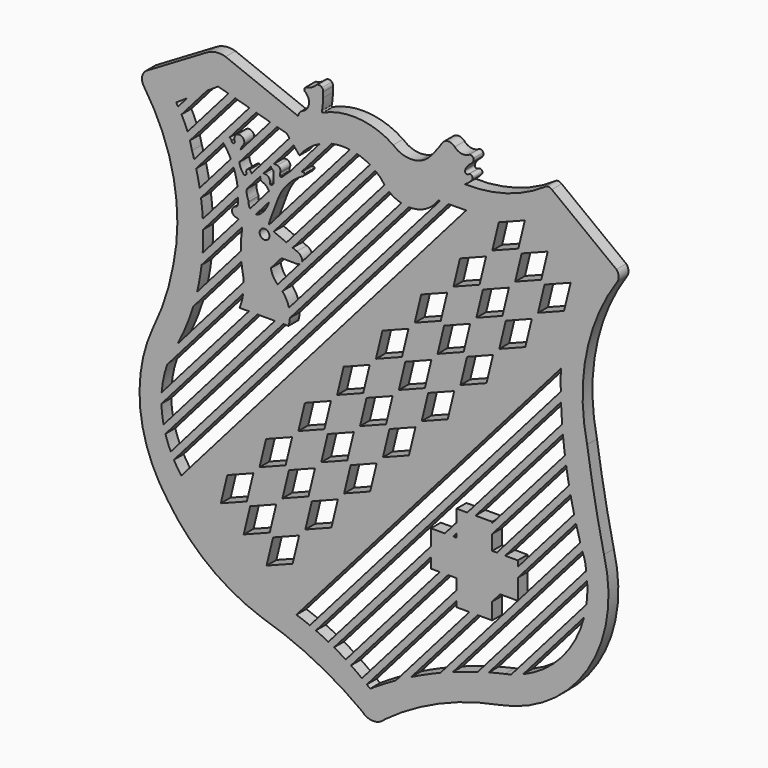
from build123d import *

# Parameters (mm, degrees)
F0_R     = 0.3088668402
F1_DEPTH = 0.77
F2_SCALE = 2.61


# Not quite as in the source:
# - ends of sketch curves that miss each other by under 0.0002 mm in the source are joined


with BuildPart() as f1:
    # F0 (on Front) → F1 (new body)
    with BuildSketch(Plane.XZ):
        with BuildLine():
            Line((-10.9450528398, 8.238459006), (-14.7752109915, 5.9727313928))
            ThreePointArc((-14.7752109915, 5.9727313928), (-15.0157556415, 5.5361442766), (-14.8831028491, 5.0556515343))
            ThreePointArc((-14.8831028491, 5.0556515343), (-13.0285590849, 0.6195466195), (-13.0580402911, -4.1885185055))
            ThreePointArc((-13.0580402911, -4.1885185055), (-13.5568964145, -6.159584329), (-14.3210859969, -8.0437213182))
            ThreePointArc((-14.3210859969, -8.0437213182), (-15.1281021661, -12.7854152226), (-13.4050389752, -17.276071012))
            ThreePointArc((-13.4050389752, -17.276071012), (-10.8401080038, -20.0274931211), (-7.5306314975, -21.8153856695))
            ThreePointArc((-7.5306314975, -21.8153856695), (-4.2408430264, -23.1051475942), (-1.226167893, -24.9484945089))
            ThreePointArc((-1.226167893, -24.9484945089), (-0.5230431925, -25.2671373593), (0.180081508, -24.9484945089))
            ThreePointArc((0.180081508, -24.9484945089), (3.5801467972, -22.973795852), (7.3375348002, -21.8153856695))
            ThreePointArc((7.3375348002, -21.8153856695), (12.9195911311, -18.040178348), (13.9394840226, -11.3789951429))
            ThreePointArc((13.9394840226, -11.3789951429), (13.3587393158, -8.5258534115), (12.8830319769, -5.6533310562))
            ThreePointArc((12.8830319769, -5.6533310562), (12.826516045, -0.6803487089), (14.7480200976, 3.9067603648))
            ThreePointArc((14.7480200976, 3.9067603648), (14.8574048465, 4.2653018977), (14.7159444168, 4.6124416403))
            Line((14.7159444168, 4.6124416403), (10.6676835567, 7.7041857041))
            ThreePointArc((10.6676835567, 7.7041857041), (10.4508174999, 7.789802789), (10.2339514432, 7.7041857041))
            ThreePointArc((10.2339514432, 7.7041857041), (7.8431577076, 6.5715789898), (5.2206409829, 6.223586627))
            Line((5.2206409829, 6.223586627), (5.2057327849, 6.2239474028))
            ThreePointArc((5.2057327849, 6.2239474028), (5.2128688846, 6.2275017661), (5.2199811789, 6.2311035281))
            ThreePointArc((5.2199811789, 6.2311035281), (5.4576814871, 6.3909100368), (5.6506660767, 6.6025618852))
            ThreePointArc((5.6506660767, 6.6025618852), (5.666017401, 6.8296722857), (5.438990331, 6.8450179774))
            ThreePointArc((5.438990331, 6.8450179774), (5.2774498824, 6.8438940146), (5.2317598398, 6.9988423926))
            ThreePointArc((5.2317598398, 6.9988423926), (5.3413345105, 7.2160766667), (5.5031483062, 7.39777321))
            ThreePointArc((5.5031483062, 7.39777321), (5.6486132018, 7.5233006308), (5.7621701773, 7.6782908968))
            ThreePointArc((5.7621701773, 7.6782908968), (5.7744494367, 7.7563651745), (5.7568072409, 7.8334049433))
            ThreePointArc((5.7568072409, 7.8334049433), (5.6517282464, 7.9393365939), (5.5027715738, 7.9479979673))
            ThreePointArc((5.5027715738, 7.9479979673), (5.0188791458, 7.8403294095), (4.5830812305, 8.0766016617))
            ThreePointArc((4.5830812305, 8.0766016617), (4.14755377, 8.2479055445), (3.7629532162, 7.9812379554))
            ThreePointArc((3.7629532162, 7.9812379554), (3.4440060295, 7.5359280459), (3.0954068061, 7.1134273894))
            ThreePointArc((3.0954068061, 7.1134273894), (2.7632061359, 6.8020403745), (2.3577139174, 6.5949287643))
            ThreePointArc((2.3577139174, 6.5949287643), (1.4977198293, 6.5400653755), (0.7303855964, 6.9322362542))
            ThreePointArc((0.7303855964, 6.9322362542), (-1.4116971773, 7.6752869671), (-3.6468112376, 7.2946189903))
            ThreePointArc((-3.6468112376, 7.2946189903), (-3.7266554182, 7.2894142265), (-3.7329988554, 7.369176019))
            ThreePointArc((-3.7329988554, 7.369176019), (-3.6863749188, 7.7291436193), (-3.6669184756, 8.0915962529))
            ThreePointArc((-3.6669184756, 8.0915962529), (-3.6669370542, 8.2476662803), (-3.6719986238, 8.4036542103))
            ThreePointArc((-3.6719986238, 8.4036542103), (-3.6744007516, 8.529985654), (-3.7354342298, 8.6406216267))
            ThreePointArc((-3.7354342298, 8.6406216267), (-3.9275077773, 8.7250033825), (-4.120208323, 8.6420634761))
            ThreePointArc((-4.120208323, 8.6420634761), (-4.3903821308, 8.4401648063), (-4.7114635818, 8.3368998021))
            ThreePointArc((-4.7114635818, 8.3368998021), (-4.8381657863, 8.2245188579), (-4.7927666456, 8.0613568425))
            ThreePointArc((-4.7927666456, 8.0613568425), (-4.5483256085, 7.5070030075), (-4.8736855388, 6.9959252141))
            ThreePointArc((-4.8736855388, 6.9959252141), (-5.1085754677, 6.8393309853), (-5.2295372828, 6.5842559561))
            Line((-5.2295372828, 6.5842559561), (-9.7806490958, 8.3812242374))
            ThreePointArc((-9.7806490958, 8.3812242374), (-10.3777742193, 8.4315567602), (-10.9450528398, 8.238459006))
        make_face()
        Polygon((-5.5775461902, -18.2294403803), (-7.2106110116, -18.8645213511), (-6.8023452719, -17.1747529548), (-5.1692804505, -16.5396719839), align=None, mode=Mode.SUBTRACT)
        Polygon((-8.4461733818, -15.7241220544), (-10.0792382032, -16.3592030252), (-9.6709724635, -14.6694346289), (-8.0379076422, -14.0343536581), align=None, mode=Mode.SUBTRACT)
        with BuildLine():
            ThreePointArc((-13.6667065556, -13.1795461358), (-13.7572572831, -12.6297862933), (-13.7985303908, -12.0741498572))
            Line((-13.7985303908, -12.0741498572), (-7.7867736006, -5.1905978471))
            Line((-7.7867736006, -5.1905978471), (-6.6895508588, -5.1905978471))
            Line((-6.6895508588, -5.1905978471), (-13.6667065556, -13.1795461358))
        make_face(mode=Mode.SUBTRACT)
        Polygon((-7.011859786, -16.9767812173), (-8.6449246074, -17.6118621881), (-8.2366588677, -15.9220937918), (-6.6035940463, -15.287012821), align=None, mode=Mode.SUBTRACT)
        Polygon((-4.5809357093, -14.1933365607), (-6.2140005306, -14.8284175315), (-5.805734791, -13.1386491352), (-4.1726699696, -12.5035681644), align=None, mode=Mode.SUBTRACT)
        Polygon((-3.1466221135, -15.4459957236), (-4.7796869348, -16.0810766945), (-4.3714211952, -14.3913082981), (-2.7383563738, -13.7562273273), align=None, mode=Mode.SUBTRACT)
        Polygon((-6.0152493051, -12.9406773977), (-7.6483141265, -13.5757583686), (-7.2400483868, -11.8859899723), (-5.6069835654, -11.2509090014), align=None, mode=Mode.SUBTRACT)
        Polygon((-3.5843252284, -10.1572327411), (-5.2173900497, -10.7923137119), (-4.80912431, -9.1025453156), (-3.1760594887, -8.4674643448), align=None, mode=Mode.SUBTRACT)
        Polygon((-2.1500116325, -11.4098919041), (-3.7830764539, -12.0449728749), (-3.3748107142, -10.3552044786), (-1.7417458929, -9.7201235077), align=None, mode=Mode.SUBTRACT)
        Polygon((-0.7156980367, -12.662551067), (-2.3487628581, -13.2976320378), (-1.9404971184, -11.6078636415), (-0.307432297, -10.9727826707), align=None, mode=Mode.SUBTRACT)
        with BuildLine():
            ThreePointArc((-1.2333306094, -23.1370316943), (-1.571815927, -22.8880537555), (-1.9174369369, -22.6490800294))
            Line((-1.9174369369, -22.6490800294), (4.1664697033, -15.6829153552))
            Line((4.1664697033, -15.6829153552), (4.6998463428, -15.6829153552))
            Line((4.6998463428, -15.6829153552), (4.6998463428, -16.3434547816))
            Line((4.6998463428, -16.3434547816), (-1.2333306094, -23.1370316943))
        make_face(mode=Mode.SUBTRACT)
        with BuildLine():
            ThreePointArc((0.8920551407, -22.5697107783), (0.0769750695, -23.0424218327), (-0.7199500254, -23.5451361219))
            ThreePointArc((-0.7199500254, -23.5451361219), (-0.8217137816, -23.4611676966), (-0.9242442608, -23.3781372242))
            Line((-0.9242442608, -23.3781372242), (4.6998463428, -16.9384688328))
            Line((4.6998463428, -16.9384688328), (4.6998463428, -17.2902317473))
            Line((4.6998463428, -17.2902317473), (5.5028932468, -17.2902317473))
            Line((5.5028932468, -17.2902317473), (0.8920551407, -22.5697107783))
        make_face(mode=Mode.SUBTRACT)
        with BuildLine():
            Line((3.6468136075, -15.6829153552), (-2.2488664966, -22.4335578124))
            ThreePointArc((-2.2488664966, -22.4335578124), (-2.6119716601, -22.2119287852), (-2.9814786804, -22.0011460831))
            Line((-2.9814786804, -22.0011460831), (3.0925299507, -15.0463147783))
            Line((3.0925299507, -15.0463147783), (3.0925299507, -15.6829153552))
            Line((3.0925299507, -15.6829153552), (3.6468136075, -15.6829153552))
        make_face(mode=Mode.SUBTRACT)
        with BuildLine():
            Line((8.5365600495, -15.6829153552), (3.6889344902, -21.2335195841))
            ThreePointArc((3.6889344902, -21.2335195841), (2.7640681021, -21.6292399404), (1.8556529669, -22.061390815))
            Line((1.8556529669, -22.061390815), (6.0225493426, -17.2902317473))
            Line((6.0225493426, -17.2902317473), (6.9292436575, -17.2902317473))
            Line((6.9292436575, -17.2902317473), (6.9292436575, -16.2520531098))
            Line((6.9292436575, -16.2520531098), (7.4263006647, -15.6829153552))
            Line((7.4263006647, -15.6829153552), (8.5365600495, -15.6829153552))
        make_face(mode=Mode.SUBTRACT)
        with BuildLine():
            ThreePointArc((12.6890300152, -15.2558443111), (11.2945144522, -17.8938182952), (8.8682408565, -19.6307054059))
            Line((8.8682408565, -19.6307054059), (12.6890300152, -15.2558443111))
        make_face(mode=Mode.SUBTRACT)
        with BuildLine():
            Line((-4.1196529229, -21.4380949639), (11.2479575195, -3.8419497037))
            ThreePointArc((11.2479575195, -3.8419497037), (11.2764123646, -4.4385333427), (11.3167625343, -5.0344306328))
            Line((11.3167625343, -5.0344306328), (5.3676957448, -11.8462016484))
            Line((5.3676957448, -11.8462016484), (4.6998463428, -11.8462016484))
            Line((4.6998463428, -11.8462016484), (4.6998463428, -12.6108992658))
            Line((4.6998463428, -12.6108992658), (3.9639444228, -13.4535180405))
            Line((3.9639444228, -13.4535180405), (3.0925299507, -13.4535180405))
            Line((3.0925299507, -13.4535180405), (3.0925299507, -14.4513007271))
            Line((3.0925299507, -14.4513007271), (-3.3360950096, -21.8121730663))
            ThreePointArc((-3.3360950096, -21.8121730663), (-3.7250476456, -21.6192138986), (-4.1196529229, -21.4380949639))
        make_face(mode=Mode.SUBTRACT)
        Polygon((4.6998463428, -13.4535180405), (4.4836005186, -13.4535180405), (4.6998463428, -13.2059133171), align=None, mode=Mode.SUBTRACT)
        with BuildLine():
            Line((-5.3373983951, -20.9661541004), (11.2354560879, -1.9899862731))
            ThreePointArc((11.2354560879, -1.9899862731), (11.2268252487, -2.6277027287), (11.2317807175, -3.2654583342))
            Line((11.2317807175, -3.2654583342), (-4.4989278267, -21.2773563861))
            ThreePointArc((-4.4989278267, -21.2773563861), (-4.9157411664, -21.1152298116), (-5.3373983952, -20.9661541004))
        make_face(mode=Mode.SUBTRACT)
        Polygon((1.71522604, -9.8791064104), (0.0821612187, -10.5141873812), (0.4904269583, -8.8244189849), (2.1234917797, -8.1893380141), align=None, mode=Mode.SUBTRACT)
        with BuildLine():
            Line((6.0321875111, -20.4167373638), (4.4722335106, -20.9316444673))
            Line((4.4722335106, -20.9316444673), (12.5894441115, -11.6373161539))
            ThreePointArc((12.5894441115, -11.6373161539), (12.7448209703, -12.1294752601), (12.8245471129, -12.6393833853))
            Line((12.8245471129, -12.6393833853), (6.0321875111, -20.4167373638))
        make_face(mode=Mode.SUBTRACT)
        with BuildLine():
            ThreePointArc((8.1273773746, -19.8839911925), (7.9218788322, -19.9370827443), (7.7147563921, -19.9834363697))
            ThreePointArc((7.7147563921, -19.9834363697), (7.2158699773, -20.0991111557), (6.7194254717, -20.2248536063))
            Line((6.7194254717, -20.2248536063), (12.8830319769, -13.1674313871))
            ThreePointArc((12.8830319769, -13.1674313871), (12.895286878, -13.8286196949), (12.8402937453, -14.4876310122))
            Line((12.8402937453, -14.4876310122), (8.1273773746, -19.8839911925))
        make_face(mode=Mode.SUBTRACT)
        with BuildLine():
            Line((8.5365600495, -14.4116516486), (12.1862088162, -10.2327488784))
            ThreePointArc((12.1862088162, -10.2327488784), (12.315988426, -10.716281355), (12.453835442, -11.1975760705))
            Line((12.453835442, -11.1975760705), (8.5464982905, -15.6715359198))
            Line((8.5464982905, -15.6715359198), (8.5365600495, -14.4116516486))
        make_face(mode=Mode.SUBTRACT)
        with BuildLine():
            Line((7.74343148, -13.4535180405), (11.8433498423, -8.7590498063))
            ThreePointArc((11.8433498423, -8.7590498063), (11.9524009398, -9.2657852479), (12.0702086391, -9.770556776))
            Line((12.0702086391, -9.770556776), (8.5365600495, -13.8166375973))
            Line((8.5365600495, -13.8166375973), (8.5365600495, -13.4535180405))
            Line((8.5365600495, -13.4535180405), (7.74343148, -13.4535180405))
        make_face(mode=Mode.SUBTRACT)
        with BuildLine():
            Line((5.8873518406, -11.8462016484), (11.3637776151, -5.5756117089))
            ThreePointArc((11.3637776151, -5.5756117089), (11.4231257209, -6.1378278281), (11.4930792726, -6.6988230715))
            Line((11.4930792726, -6.6988230715), (6.9292436575, -11.9244835428))
            Line((6.9292436575, -11.9244835428), (6.9292436575, -11.8462016484))
            Line((6.9292436575, -11.8462016484), (5.8873518406, -11.8462016484))
        make_face(mode=Mode.SUBTRACT)
        with BuildLine():
            Line((6.9292436575, -12.5194975941), (11.5669223234, -7.2146120887))
            ThreePointArc((11.5669223234, -7.2146120887), (11.6524503811, -7.7450187223), (11.7474826057, -8.2738051838))
            Line((11.7474826058, -8.2738051838), (7.2237753842, -13.4535180405))
            Line((7.2237753842, -13.4535180405), (6.9292436575, -13.4535180405))
            Line((6.9292436575, -13.4535180405), (6.9292436575, -12.5194975941))
        make_face(mode=Mode.SUBTRACT)
        with BuildLine():
            ThreePointArc((-13.7858184066, -11.4496532401), (-13.6697387353, -10.6130173489), (-13.4420062366, -9.7996465765))
            Line((-13.4420062366, -9.7996465765), (-8.677906045, -4.3446801508))
            ThreePointArc((-8.677906045, -4.3446801508), (-8.7616198951, -4.7738576747), (-8.8940169662, -5.1905978471))
            Line((-8.8940169662, -5.1905978471), (-8.3194663395, -5.1905978471))
            Line((-8.3194663395, -5.1905978471), (-13.7858184066, -11.4496532401))
        make_face(mode=Mode.SUBTRACT)
        with BuildLine():
            Line((-8.6455751358, -3.6977195694), (-12.77777931, -8.4291555443))
            ThreePointArc((-12.77777931, -8.4291555443), (-12.2372024074, -7.2658242862), (-11.8043741052, -6.0582553795))
            Line((-11.8043741052, -6.0582553795), (-8.7869307107, -2.6032372762))
            ThreePointArc((-8.7869307107, -2.6032372762), (-8.7410410218, -2.9675427525), (-8.6765894666, -3.32902628))
            ThreePointArc((-8.6765894666, -3.32902628), (-8.656598502, -3.5129957493), (-8.6455751358, -3.6977195694))
        make_face(mode=Mode.SUBTRACT)
        with BuildLine():
            Line((-8.821167106, -2.0324972603), (-11.5625482211, -5.1714198987))
            ThreePointArc((-11.5625482211, -5.1714198987), (-11.3989515702, -4.3856405891), (-11.2802423771, -3.5918389041))
            Line((-11.2802423771, -3.5918389041), (-8.7387201501, -0.6817577008))
            ThreePointArc((-8.7387201501, -0.6817577008), (-8.7348520945, -0.7841341496), (-8.7522082031, -0.8851027815))
            ThreePointArc((-8.7522082031, -0.8851027815), (-8.8096825125, -1.45741802), (-8.821167106, -2.0324972603))
        make_face(mode=Mode.SUBTRACT)
        with BuildLine():
            Line((-8.9664455479, -0.3325655051), (-11.2144849522, -2.906604459))
            ThreePointArc((-11.2144849522, -2.906604459), (-11.1831679624, -2.2599358856), (-11.1815104167, -1.6125115655))
            Line((-11.1815104167, -1.6125115655), (-8.9905998315, 0.8961140307))
            ThreePointArc((-8.9905998315, 0.8961140307), (-8.9944051774, 0.699791789), (-9.0069510043, 0.5038338713))
            ThreePointArc((-9.0069510043, 0.5038338713), (-9.0500825749, 0.3900487183), (-9.1431997716, 0.3117123852))
            ThreePointArc((-9.1431997716, 0.3117123852), (-9.3792556973, 0.0232370221), (-9.1431997716, -0.2652383409))
            ThreePointArc((-9.1431997716, -0.2652383409), (-9.0515665528, -0.2903536547), (-8.9664455479, -0.3325655051))
        make_face(mode=Mode.SUBTRACT)
        with BuildLine():
            ThreePointArc((1.7099666153, 3.8170348811), (2.7552211547, 4.0603120463), (3.5440460779, 4.7879768535))
            Line((3.5440460779, 4.7879768535), (3.6562696517, 4.7892445983))
            Line((3.6562696517, 4.7892445983), (-13.2163624103, -14.530173069))
            ThreePointArc((-13.2163624103, -14.530173069), (-13.3983587519, -14.0977583157), (-13.5474350163, -13.6529196318))
            Line((-13.5474350163, -13.6529196318), (-6.1568581199, -5.1905978471))
            Line((-6.1568581199, -5.1905978471), (-5.8320215903, -5.1905978471))
            ThreePointArc((-5.8320215903, -5.1905978471), (-5.776941597, -4.9609351068), (-5.7512427417, -4.726162134))
            Line((-5.7512427417, -4.726162134), (1.7099666152, 3.8170348811))
        make_face(mode=Mode.SUBTRACT)
        Polygon((0.2809124442, -8.6264472474), (-1.3521523772, -9.2615282183), (-0.9438866375, -7.5717598219), (0.6891781839, -6.9366788511), align=None, mode=Mode.SUBTRACT)
        Polygon((-1.1534011516, -7.3737880845), (-2.786465973, -8.0088690553), (-2.3782002333, -6.319100659), (-0.7451354119, -5.6840196882), align=None, mode=Mode.SUBTRACT)
        with BuildLine():
            Line((4.1942702487, 4.7953221758), (5.3024259397, 4.8078405671))
            Line((5.3024259397, 4.8078405671), (-12.5536639243, -15.6376510859))
            ThreePointArc((-12.5536639243, -15.6376510859), (-12.7994138666, -15.2846778771), (-13.0203282218, -14.9156521763))
            Line((-13.0203282218, -14.9156521763), (4.1942702487, 4.7953221757))
        make_face(mode=Mode.SUBTRACT)
        with BuildLine():
            ThreePointArc((-5.3103477694, -1.5955877025), (-5.2219482409, -1.5838979912), (-5.1396257073, -1.5496324623))
            Line((-5.1396257073, -1.5496324623), (-6.5157890588, -3.1253602129))
            ThreePointArc((-6.5157890588, -3.1253602129), (-6.7925168449, -2.7769712998), (-6.9431105034, -2.3583131429))
            Line((-6.9431105034, -2.3583131429), (-6.2769835025, -1.5955877025))
            Line((-6.2769835025, -1.5955877025), (-5.3103477694, -1.5955877025))
        make_face(mode=Mode.SUBTRACT)
        with Locations((-7.3358300142, -0.6240997463)):
            Circle(F0_R, mode=Mode.SUBTRACT)
        with BuildLine():
            Line((-6.2213819192, -3.3982008105), (0.4723535183, 4.2662270152))
            ThreePointArc((0.4723535183, 4.2662270152), (0.8351019863, 4.0365421249), (1.2369614373, 3.8853780368))
            Line((1.2369614373, 3.8853780368), (-5.806860176, -4.1799037295))
            ThreePointArc((-5.806860176, -4.1799037295), (-5.9672312159, -3.7641875109), (-6.2213819192, -3.3982008105))
        make_face(mode=Mode.SUBTRACT)
        with BuildLine():
            Line((-9.0287771642, 1.462341614), (-11.2054048948, -1.0299298988))
            ThreePointArc((-11.2054048948, -1.0299298988), (-11.2515233726, -0.4663115305), (-11.3201605587, 0.0950096929))
            Line((-11.3201605587, 0.0950096929), (-9.2738834577, 2.4380277728))
            ThreePointArc((-9.2738834577, 2.4380277728), (-9.1234016365, 1.9572007752), (-9.0287771642, 1.462341614))
        make_face(mode=Mode.SUBTRACT)
        with BuildLine():
            Line((-9.4511744684, 2.8449681009), (-11.403304677, 0.6097496298))
            ThreePointArc((-11.403304677, 0.6097496298), (-11.5038968619, 1.1142592273), (-11.6227900858, 1.6147720873))
            Line((-11.6227900858, 1.6147720873), (-9.9194663882, 3.5651033584))
            ThreePointArc((-9.9194663882, 3.5651033584), (-9.8876871694, 3.5294173714), (-9.8507292569, 3.4991267603))
            ThreePointArc((-9.8507292569, 3.4991267603), (-9.6367038105, 3.180750025), (-9.4511744684, 2.8449681009))
        make_face(mode=Mode.SUBTRACT)
        with BuildLine():
            ThreePointArc((-7.6002883494, 2.4880416038), (-7.6052085516, 2.4054318662), (-7.586508058, 2.3248163052))
            ThreePointArc((-7.586508058, 2.3248163052), (-7.5300428081, 2.2470948729), (-7.4444068596, 2.2035583388))
            ThreePointArc((-7.4444068596, 2.2035583388), (-7.2156162773, 2.0670054322), (-7.0590861949, 1.8513896626))
            Line((-7.0590861949, 1.8513896626), (-8.2393287905, 0.4999941263))
            ThreePointArc((-8.2393287905, 0.4999941263), (-8.3203633582, 0.6616015237), (-8.3359489217, 0.8417143836))
            ThreePointArc((-8.3359489217, 0.8417143836), (-8.3399816981, 0.9073115392), (-8.3697615191, 0.9658983327))
            ThreePointArc((-8.3697615191, 0.9658983327), (-8.4487246819, 1.2382410161), (-8.4441880507, 1.5217637441))
            Line((-8.4441880507, 1.5217637441), (-7.6002883494, 2.4880416038))
        make_face(mode=Mode.SUBTRACT)
        with BuildLine():
            ThreePointArc((-11.7503894503, 2.0786100981), (-11.8158208032, 2.2951178794), (-11.8847098202, 2.5105504319))
            ThreePointArc((-11.8847098202, 2.5105504319), (-11.9452123139, 2.7718492995), (-12.0163068847, 3.0304671874))
            Line((-12.0163068847, 3.0304671874), (-9.1722211492, 6.286988162))
            Line((-9.1722211492, 6.286988162), (-8.2881833288, 6.0428882182))
            Line((-8.2881833288, 6.0428882182), (-11.7503894503, 2.0786100981))
        make_face(mode=Mode.SUBTRACT)
        with BuildLine():
            Line((-12.1938881701, 5.3033529044), (-12.7545015611, 4.6614421337))
            ThreePointArc((-12.7545015611, 4.6614421337), (-12.8159657163, 4.7573246352), (-12.8790792078, 4.8521296121))
            Line((-12.8790792078, 4.8521296121), (-12.1938881701, 5.3033529044))
        make_face(mode=Mode.SUBTRACT)
        with BuildLine():
            Line((-10.9367561123, 6.1312202214), (-10.2488128468, 6.5842559561))
            Line((-10.2488128468, 6.5842559561), (-9.6014143384, 6.4054967042))
            Line((-9.6014143384, 6.4054967042), (-12.1642353754, 3.4710280428))
            ThreePointArc((-12.1642353754, 3.4710280428), (-12.3383105154, 3.8900821354), (-12.5408363452, 4.296150818))
            Line((-12.5408363452, 4.296150818), (-10.9400997477, 6.1290183156))
            Line((-10.9400997477, 6.1290183156), (-10.9367561123, 6.1312202214))
        make_face(mode=Mode.SUBTRACT)
        with BuildLine():
            Line((-9.5260808583, 4.015535711), (-7.8589901396, 5.9243796761))
            Line((-7.8589901396, 5.9243796761), (-6.9749523192, 5.6802797323))
            Line((-6.9749523192, 5.6802797323), (-8.8671884793, 3.5136408482))
            ThreePointArc((-8.8671884793, 3.5136408482), (-8.7699312883, 3.7246411604), (-8.6364932358, 3.9148367941))
            ThreePointArc((-8.6364932358, 3.9148367941), (-8.8043998527, 4.3404838292), (-9.215648286, 4.1398778558))
            ThreePointArc((-9.215648286, 4.1398778558), (-9.2370991293, 4.027357325), (-9.215648286, 3.9148367941))
            ThreePointArc((-9.215648286, 3.9148367941), (-9.2769327358, 3.7652720149), (-9.3970997259, 3.8733705878))
            ThreePointArc((-9.3970997259, 3.8733705878), (-9.4501275498, 3.9548528695), (-9.5260808583, 4.015535711))
        make_face(mode=Mode.SUBTRACT)
        with BuildLine():
            ThreePointArc((-7.0583481676, 1.2422935111), (-7.3031784221, 0.7325767375), (-7.7065480873, 0.3362864954))
            ThreePointArc((-7.7065480873, 0.3362864954), (-7.7876341449, 0.316983455), (-7.870836, 0.3119827138))
            Line((-7.870836, 0.3119827138), (-7.0583481676, 1.2422935111))
        make_face(mode=Mode.SUBTRACT)
        with BuildLine():
            ThreePointArc((-6.8379025906, 3.1115673482), (-6.7799474463, 3.0419714884), (-6.7711481825, 2.9518329538))
            Line((-6.7711481825, 2.9518329538), (-6.7711481825, 2.410643734))
            ThreePointArc((-6.7711481825, 2.410643734), (-6.8282876064, 2.2823449264), (-6.9618755952, 2.2389888763))
            ThreePointArc((-6.9618755952, 2.2389888763), (-6.9910543822, 2.2665913301), (-7.0000211708, 2.3057435174))
            ThreePointArc((-7.0000211708, 2.3057435174), (-7.0374330915, 2.5523292397), (-7.2336625308, 2.7062713634))
            ThreePointArc((-7.2336625308, 2.7062713634), (-7.3237397741, 2.7185773587), (-7.4131814005, 2.7022818765))
            Line((-7.4131814005, 2.7022818765), (-6.9346278915, 3.2502328472))
            ThreePointArc((-6.9346278915, 3.2502328472), (-6.9058558657, 3.1672347731), (-6.8379025906, 3.1115673482))
        make_face(mode=Mode.SUBTRACT)
        with BuildLine():
            Line((-6.5457591299, 5.5617711901), (-5.9505729005, 5.3974287584))
            Line((-5.9505729005, 5.3974287584), (-5.7755220798, 5.1873676516))
            Line((-5.7755220798, 5.1873676516), (-8.1466662461, 2.4723718921))
            ThreePointArc((-8.1466662461, 2.4723718921), (-8.1996710185, 2.5685930795), (-8.2735326141, 2.6499102823))
            ThreePointArc((-8.2735326141, 2.6499102823), (-8.4436045696, 2.5889674414), (-8.4761111066, 2.4112546816))
            ThreePointArc((-8.4761111066, 2.4112546816), (-8.5202582261, 2.2564351573), (-8.6765894666, 2.2948876802))
            ThreePointArc((-8.6765894666, 2.2948876802), (-8.8306064216, 2.5546289938), (-8.9201967831, 2.8430043387))
            Line((-8.9201967831, 2.8430043387), (-6.5457591299, 5.5617711901))
        make_face(mode=Mode.SUBTRACT)
        with BuildLine():
            ThreePointArc((-3.127071564, 5.7436643934), (-2.5605439608, 5.8146750507), (-1.9901558077, 5.7891134924))
            Line((-1.9901558077, 5.7891134924), (-7.0597094267, -0.0156017051))
            Line((-7.0597094267, -0.0156017051), (-7.0565943606, 0.0848966592))
            ThreePointArc((-7.0565943606, 0.0848966592), (-7.0278260356, 0.178519651), (-6.9953873753, 0.2709350957))
            Line((-6.9953873753, 0.2709350957), (-6.5143329272, 1.559508557))
            ThreePointArc((-6.5143329272, 1.559508557), (-6.3313097806, 1.965538127), (-6.096295783, 2.3438579717))
            Line((-6.096295783, 2.3438579717), (-5.6724169914, 2.829205568))
            ThreePointArc((-5.6724169914, 2.829205568), (-5.3692555434, 3.0836489297), (-5.0383298658, 3.3007583115))
            ThreePointArc((-5.0383298658, 3.3007583115), (-4.9029711292, 3.3879204261), (-4.8223878257, 3.5272960085))
            ThreePointArc((-4.8223878257, 3.5272960085), (-4.840712285, 3.5817791905), (-4.8962947913, 3.5964348353))
            ThreePointArc((-4.8962947913, 3.5964348353), (-4.9511315633, 3.5953957011), (-5.0058953666, 3.5923828604))
            Line((-5.0058953666, 3.5923828604), (-3.127071564, 5.7436643934))
        make_face(mode=Mode.SUBTRACT)
        with BuildLine():
            ThreePointArc((-5.1486627199, 4.4351359829), (-4.5819973475, 5.0381995036), (-3.8855484348, 5.4851381639))
            Line((-3.8855484348, 5.4851381639), (-5.7873457801, 3.3075515789))
            ThreePointArc((-5.7873457801, 3.3075515789), (-5.8864101461, 3.2294689096), (-5.9786736965, 3.1434567645))
            ThreePointArc((-5.9786736965, 3.1434567645), (-6.1011433537, 3.0241752891), (-6.2251905911, 2.9065352865))
            ThreePointArc((-6.2251905911, 2.9065352865), (-6.2943294179, 2.8728812457), (-6.3634682447, 2.9065352865))
            ThreePointArc((-6.3634682447, 2.9065352865), (-6.3805909303, 2.9947467847), (-6.3634682447, 3.0829582829))
            ThreePointArc((-6.3634682447, 3.0829582829), (-6.3614530323, 3.3037003101), (-6.5327389166, 3.4429563675))
            ThreePointArc((-6.5327389166, 3.4429563675), (-6.6542917607, 3.4551916182), (-6.7745268501, 3.4335509494))
            Line((-6.7745268501, 3.4335509494), (-5.5154209678, 4.875246136))
            Line((-5.5154209678, 4.875246136), (-5.1486627199, 4.4351359829))
        make_face(mode=Mode.SUBTRACT)
        with BuildLine():
            ThreePointArc((-0.395993089, 5.1382348379), (-0.1911236911, 4.9708761253), (0, 4.7879768535))
            ThreePointArc((0, 4.7879768535), (0.0865355453, 4.6625062507), (0.1819379724, 4.5436380478))
            Line((0.1819379724, 4.5436380478), (-4.99591019, -1.3850760318))
            ThreePointArc((-4.99591019, -1.3850760318), (-4.9794877489, -1.3341949744), (-4.9712425098, -1.2813688955))
            ThreePointArc((-4.9712425098, -1.2813688955), (-5.0880391236, -1.0454539409), (-5.3103477694, -0.9044710314))
            Line((-5.3103477694, -0.9044710314), (-5.5750850123, -0.7919033667))
            Line((-5.5750850123, -0.7919033667), (-0.395993089, 5.1382348379))
        make_face(mode=Mode.SUBTRACT)
        with BuildLine():
            ThreePointArc((-1.5369210948, 5.6981328566), (-1.1242035733, 5.5561071097), (-0.7332814788, 5.3619757587))
            Line((-0.7332814788, 5.3619757587), (-5.963528089, -0.6267353324))
            Line((-5.963528089, -0.6267353324), (-6.7636301865, -0.2865277226))
            Line((-6.7636301865, -0.2865277226), (-1.5369210948, 5.6981328566))
        make_face(mode=Mode.SUBTRACT)
        Polygon((4.1461501168, -7.0956617538), (2.5130852954, -7.7307427246), (2.9213510351, -6.0409743283), (4.5544158564, -5.4058933574), align=None, mode=Mode.SUBTRACT)
        Polygon((1.2775229251, -4.5903434279), (-0.3555418962, -5.2254243987), (0.0527238434, -3.5356560024), (1.6857886648, -2.9005750316), align=None, mode=Mode.SUBTRACT)
        Polygon((2.7118365209, -5.8430025908), (1.0787716996, -6.4780835616), (1.4870374393, -4.7883151653), (3.1201022606, -4.1532341945), align=None, mode=Mode.SUBTRACT)
        Polygon((3.7084470019, -1.8068987713), (2.0753821805, -2.4419797421), (2.4836479202, -0.7522113458), (4.1167127415, -0.1171303749), align=None, mode=Mode.SUBTRACT)
        Polygon((5.1427605977, -3.0595579342), (3.5096957763, -3.694638905), (3.917961516, -2.0048705087), (5.5510263374, -1.3697895379), align=None, mode=Mode.SUBTRACT)
        Polygon((6.5770741935, -4.3122170971), (4.9440093721, -4.947298068), (5.3522751118, -3.2575296716), (6.9853399332, -2.6224487008), align=None, mode=Mode.SUBTRACT)
        Polygon((9.0079982702, -1.5287724405), (7.3749334489, -2.1638534113), (7.7831991886, -0.474085015), (9.4162640099, 0.1609959558), align=None, mode=Mode.SUBTRACT)
        Polygon((7.5736846744, -0.2761132776), (5.9406198531, -0.9111942484), (6.3488855927, 0.7785741479), (7.9819504141, 1.4136551187), align=None, mode=Mode.SUBTRACT)
        Polygon((6.1393710786, 0.9765458854), (4.5063062572, 0.3414649145), (4.9145719969, 2.0312333109), (6.5476368183, 2.6663142817), align=None, mode=Mode.SUBTRACT)
        Polygon((11.438922347, 1.2546722161), (9.8058575256, 0.6195912453), (10.2141232653, 2.3093596416), (11.8471880867, 2.9444406124), align=None, mode=Mode.SUBTRACT)
        Polygon((8.5702951554, 3.759990542), (6.937230334, 3.1249095712), (7.3454960737, 4.8146779675), (8.978560895, 5.4497589383), align=None, mode=Mode.SUBTRACT)
        Polygon((10.0046087512, 2.5073313791), (8.3715439298, 1.8722504082), (8.7798096695, 3.5620188045), (10.4128744908, 4.1970997754), align=None, mode=Mode.SUBTRACT)
    extrude(amount=F1_DEPTH)


with BuildPart() as f1_1:
    # F2: moved
    add(f1.part.scale(F2_SCALE))


solid = f1_1.part
